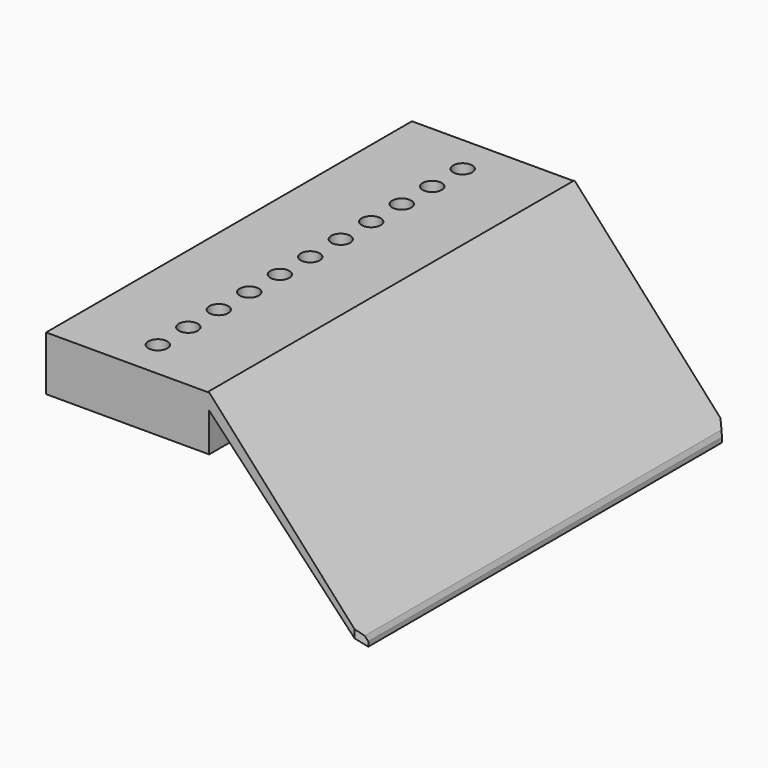
from build123d import *

# Parameters (mm, degrees)
F0_W        = 108.7058566231
F0_H        = 36.235285541
F1_DEPTH    = 304.8
F3_DEPTH    = 304.8
F4_T1_DEPTH = 31.2448363711
F4_T3_DEPTH = 315.5177056065
F6_D        = 12.7


# Not quite as in the source:
# - a fillet or chamfer that OpenCascade refuses, or shapes differently, is made with other operations: its cross-section is extruded or revolved along the edge and cut away or added
# - a feature names something its author has since deleted; it is built from what else it names


with BuildPart() as f1:
    # F0 (on Front) → F1 (new body)
    with BuildSketch(Plane.XZ):
        with Locations((54.3529283115, 18.1176427705)):
            Rectangle(F0_W, F0_H)
    extrude(amount=-F1_DEPTH)

    # F2 (on face) → F3 (join)
    with BuildSketch(Plane.XZ):
        Polygon((210.6682882407, -76.6480192542), (108.3266659877, 36.8101285866), (108.3266659877, 36.235285541), (108.7058566231, 36.235285541), (108.7058566231, 25.7386137456), (210.6682882407, -81.7645564675), align=None)
    extrude(amount=-F3_DEPTH)

    # F4: chamfer of 5.08 on 3 edges, made by hand

    # F4_s2 → F4_t1 (cut)
    with BuildSketch(Plane.XY.offset(-94.8287060464)):
        Polygon((205.5882882407, 0), (210.6682882407, 5.08), (210.6682882407, 0), align=None)
        Polygon((205.5882882407, 304.8), (210.6682882407, 299.72), (210.6682882407, 304.8), align=None)
    extrude(amount=F4_T1_DEPTH, mode=Mode.SUBTRACT)

    # F4_s4 → F4_t3 (cut)
    with BuildSketch(Plane.XZ.offset(-310.1588528033)):
        Polygon((209.3604296259, -75.1980987546), (210.6682882407, -78.6006491759), (210.6682882407, -76.6480192542), align=None)
    extrude(amount=F4_T3_DEPTH, mode=Mode.SUBTRACT)

    # F6 (through all)
    with Locations(Plane.XY.offset(36.235285541)):
        with Locations((54.1633329939, 228.6), (54.1633329939, 152.4), (54.1633329939, 279.4), (54.1633329939, 254), (54.1633329939, 177.8), (54.1633329939, 203.1635642052), (54.1633329939, 127.0884871483), (54.1633329939, 101.6), (54.1633329939, 50.8), (54.1633329939, 25.4), (54.1633329939, 76.2)):
            Hole(F6_D / 2)


solid = f1.part
